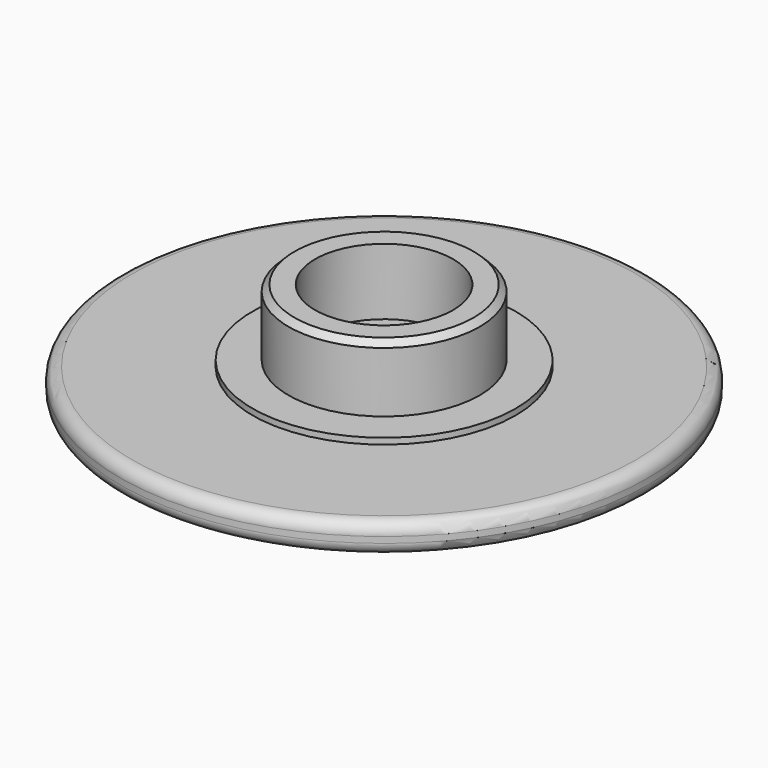
from build123d import *

# Parameters (mm, degrees)
F0_R         = 11.1125
F1_DEPTH     = 1.27
F2_R         = 4.0259
F2_R_2       = 2.9047174061
F3_DEPTH     = 3.048
F4_R         = 5.5397216457
F5_DEPTH     = 0.254
F6_R         = 0.508
F7_SIZE      = 0.254
F8_TEXT_SIZE = 14.1111111111
F9_DEPTH     = 0.508


# Not quite as in the source:
# - Text() gives the source's letters only with a copy of the font that has no kerning and outlines rounded to 1/6400 em; it was checked with that copy


with BuildPart() as f1:
    # F0 (on Top) → F1 (new body)
    with BuildSketch(Plane.XY):
        Circle(F0_R)
    extrude(amount=F1_DEPTH)

    # F2 (on face) → F3 (join)
    with BuildSketch(Plane.XY.offset(1.27)):
        Circle(F2_R)
        Circle(F2_R_2, mode=Mode.SUBTRACT)
    extrude(amount=F3_DEPTH)

    # F4 (on face) → F5 (join)
    with BuildSketch(Plane.XY.offset(1.27)):
        Circle(F4_R)
    extrude(amount=F5_DEPTH)

    # F6
    f6_edges = [f1.edges().sort_by_distance(p)[0] for p in [
        (11.1125, 0, 0.635),
        (-11.1125, 0, 0),
        (-11.1125, 0, 1.27),
    ]]
    fillet(f6_edges, radius=F6_R)

    # F7
    f7_edges = [f1.edges().sort_by_distance(p)[0] for p in [
        (-4.0259, 0, 4.318),
    ]]
    chamfer(f7_edges, length=F7_SIZE)

    # F8 (on face) → F9 (cut)
    with BuildSketch(Plane(origin=(0, 0, 0), x_dir=(1, 0, 0), z_dir=(0, 0, -1))):
        with Locations((-5.8684809448, -5.011664038)):
            Text('EJ', F8_TEXT_SIZE, font='Open Sans', text_align=(TextAlign.LEFT, TextAlign.BOTTOM))
    extrude(amount=-F9_DEPTH, mode=Mode.SUBTRACT)


solid = f1.part
